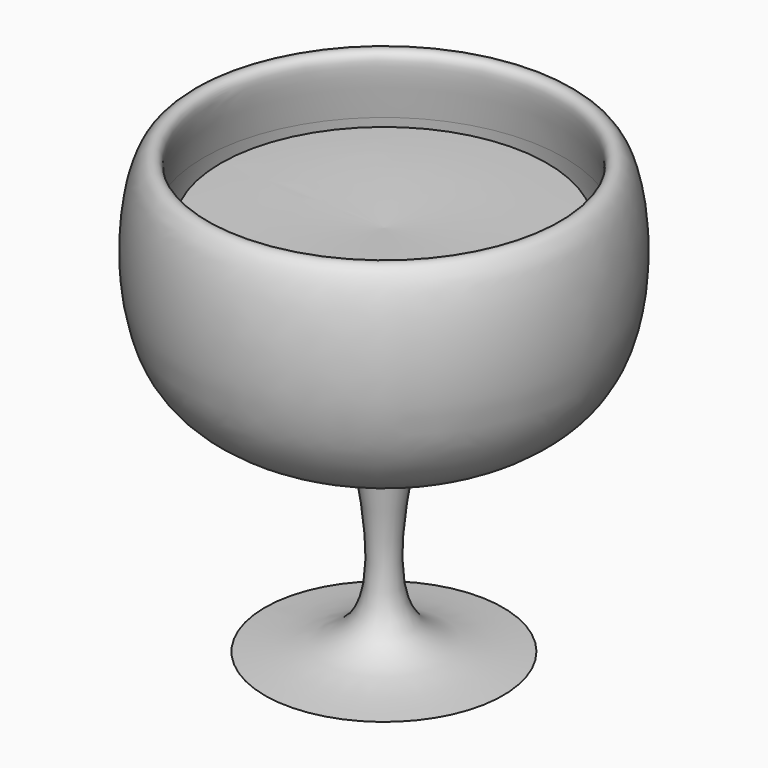
from build123d import *


with BuildPart() as f1:
    # F0 (on Front) → F1 (revolve)
    with BuildSketch(Plane.XZ):
        with BuildLine():
            Line((-30.2555859089, 0), (0, 0))
            Line((0, 0), (0, 52.856143564))
            add(Edge.make_bspline(
                [(-45.7740813332, 95.6038505465), (-47.2095188305, 87.2991599033), (-50.3677045823, 59.6871122056), (-19.4256343902, 55.4906868783), (0, 52.856143564)],
                knots=[0.6387837514, 0.6387837514, 0.6387837514, 0.6387837514, 0.7732260726, 1, 1, 1, 1], degree=3))
            add(Edge.make_bspline(
                [(-6.5614529885, 46.2946929038), (-23.7375813703, 49.7656176795), (-57.2711940094, 56.5420369251), (-52.1380161092, 111.1924627948), (-43.8581904367, 111.4959441101), (-43.5443703874, 106.9256896786), (-45.1418815845, 99.2614276595), (-45.7740813332, 95.6038505465)],
                knots=[0, 0, 0, 0, 0.2235059953, 0.4363593065, 0.5002150277, 0.5795722554, 0.6387837514, 0.6387837514, 0.6387837514, 0.6387837514], degree=3))
            add(Edge.make_bspline(
                [(-30.2555859089, 0), (-20.7758611956, 0.8405917515), (0.596171045, 2.7357052234), (-4.0025365403, 30.7219540283), (-6.5614529885, 46.2946929038)],
                knots=[0, 0, 0, 0, 0.4435574777, 1, 1, 1, 1], degree=3))
        make_face()
    revolve(axis=Axis((0, 0, 73.816338554), (0, 0, 1)))


with BuildPart() as f1b:
    # F0 (on Front) → F1, piece 2 (revolve)
    with BuildSketch(Plane.XZ):
        with BuildLine():
            Line((-1.8814868527, 57.6472505927), (0, 93.0105522275))
            Line((0, 93.0105522275), (0, 94.7765335441))
            add(Edge.make_bspline(
                [(-41.4458089809, 95.732617781), (-38.525826684, 95.8117367036), (-30.6747257433, 95.9659891353), (-16.2903872548, 95.5532858195), (-5.4474588845, 95.0359859374), (0, 94.7765335441)],
                knots=[0.1035632862, 0.1035632862, 0.1035632862, 0.1035632862, 0.3118574773, 0.6539330232, 1, 1, 1, 1], degree=3))
            Line((-41.4458089809, 95.732617781), (-41.4458089809, 75.3289014101))
            Line((-41.4458089809, 75.3289014101), (-28.4897945821, 64.5139068365))
            Line((-28.4897945821, 64.5139068365), (-1.8814868527, 57.6472505927))
        make_face()
    revolve(axis=Axis((0, 0, 73.816338554), (0, 0, 1)))


solid = Compound([f1.part, f1b.part])
